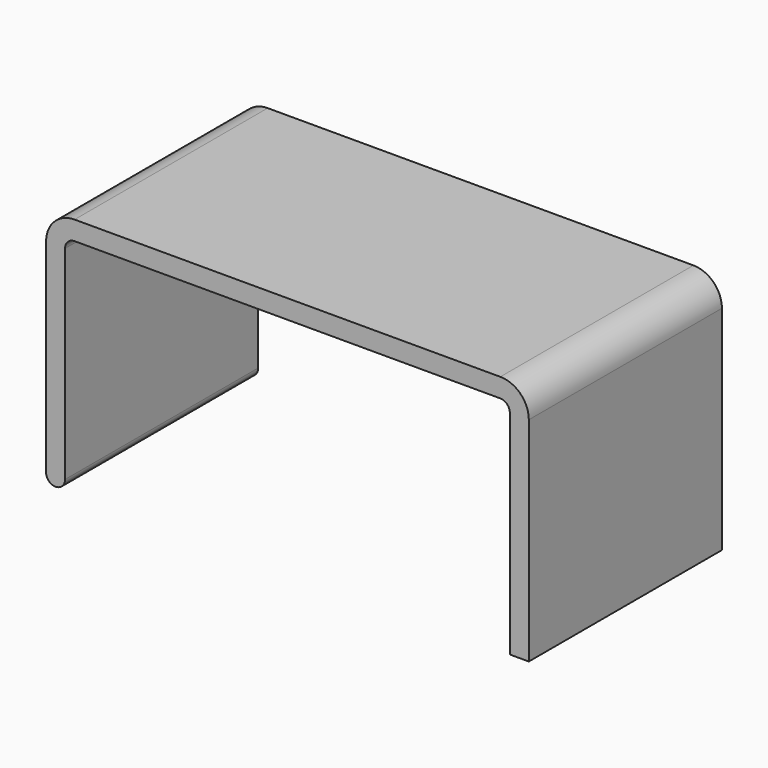
from build123d import *

# Parameters (mm, degrees)
F0_W     = 50.8
F0_H     = 25.4
F1_DEPTH = 12.7
F2_W     = 46.8
F2_H     = 23.4
F3_DEPTH = 25.4
F4_R     = 3
F5_R     = 1
F6_R     = 0.99999


# Not quite as in the source:
# - a fillet or chamfer is up to 0.001 mm smaller than in the source, because OpenCascade refuses the exact size


with BuildPart() as f1:
    # F0 (on Front) → F1 (new body, symmetric)
    with BuildSketch(Plane.XZ):
        Rectangle(F0_W, F0_H)
    extrude(amount=F1_DEPTH, both=True)

    # F2 (on face) → F3 (cut, through all)
    with BuildSketch(Plane.XZ.offset(12.7)):
        with Locations((0, -1)):
            Rectangle(F2_W, F2_H)
    extrude(amount=-F3_DEPTH, mode=Mode.SUBTRACT)

    # F4
    f4_edges = [f1.edges().sort_by_distance(p)[0] for p in [
        (-25.4, 0, 12.7),
        (25.4, 0, 12.7),
    ]]
    fillet(f4_edges, radius=F4_R)

    # F5
    f5_edges = [f1.edges().sort_by_distance(p)[0] for p in [
        (-23.4, 0, 10.7),
        (23.4, 0, 10.7),
    ]]
    fillet(f5_edges, radius=F5_R)

    # F6 (radius 1 in the source; OpenCascade refuses exactly that, so slightly less here)
    f6_edges = [f1.edges().sort_by_distance(p)[0] for p in [
        (-25.4, 0, -12.7),
        (-23.4, 0, -12.7),
    ]]
    fillet(f6_edges, radius=F6_R)


solid = f1.part
